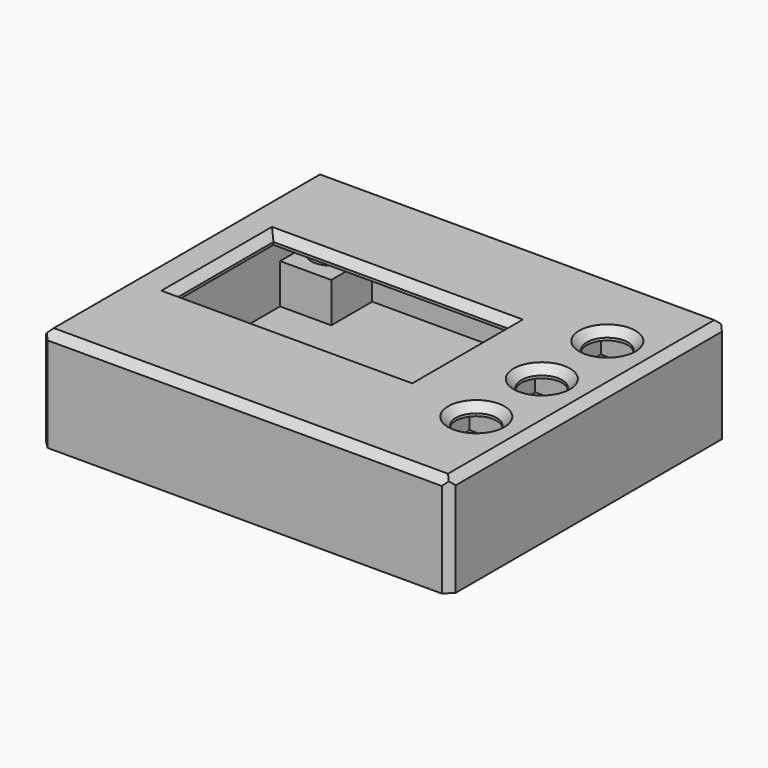
from build123d import *

# Parameters (mm, degrees)
F0_W      = 40
F0_H      = 34
F1_DEPTH  = 10
F2_W      = 37.9
F2_H      = 31.9
F3_DEPTH  = 9
F4_R      = 2
F4_W      = 23
F4_H      = 12
F5_DEPTH  = 25
F6_W      = 6.4
F6_H      = 6.4
F7_DEPTH  = 2.5
F6_W_2    = 5
F6_H_2    = 3.5
F8_DEPTH  = 1.5
F9_DEPTH  = 4
F10_R     = 1.05
F11_DEPTH = 2
F12_SIZE  = 0.75
F14_DEPTH = 2.5
F15_W     = 2
F15_H     = 2.5
F16_DEPTH = 1.1
F17_SIZE  = 0.75
F18_W     = 4.5
F18_H     = 3.5
F19_W     = 4.5
F19_H     = 3.5
F20_DEPTH = 5
F21_W     = 4.5
F21_H     = 3.5
F22_DEPTH = 4
F23_R     = 1.05
F24_R     = 1.05
F25_R     = 1.05
F26_DEPTH = 4
F27_W     = 37.5
F27_H     = 31.5
F28_DEPTH = 1.05
F29_W     = 18.5
F29_H     = 2.5
F30_DEPTH = 25
F32_R     = 1.05
F33_DEPTH = 2.95
F31_R     = 1.05
F34_DEPTH = 2.95
F35_R     = 1.05
F36_DEPTH = 2.95
F38_START = 1.6
F37_R     = 1.05
F38_DEPTH = 4.85
F39_W     = 5
F39_H     = 5
F40_DEPTH = 2
F41_W     = 5
F41_H     = 5
F42_DEPTH = 1.9
F43_DEPTH = 25
F44_R     = 1.05
F45_DEPTH = 2.1
F46_W     = 18.5
F46_H     = 1.5
F47_DEPTH = 1.5


with BuildPart() as f1:
    # F0 (on Top) → F1 (new body)
    with BuildSketch(Plane.XY):
        Rectangle(F0_W, F0_H)
    extrude(amount=F1_DEPTH)

    # F2 (on face) → F3 (cut)
    with BuildSketch(Plane(origin=(0, 0, 0), x_dir=(1, 0, 0), z_dir=(0, 0, -1))):
        Rectangle(F2_W, F2_H)
    extrude(amount=-F3_DEPTH, mode=Mode.SUBTRACT)

    # F4 (on face) → F5 (cut)
    with BuildSketch(Plane.XY.offset(10)):
        with Locations((15.05, -7.55)):
            Circle(F4_R)
        with Locations((15.05, 0.45)):
            Circle(F4_R)
        with Locations((15.05, 8.45)):
            Circle(F4_R)
        with Locations((-4.45, 0.45)):
            Rectangle(F4_W, F4_H)
    extrude(amount=-F5_DEPTH, mode=Mode.SUBTRACT)

    # F6 (on face) → F7 (join)
    with BuildSketch(Plane(origin=(0, 0, 9), x_dir=(1, 0, 0), z_dir=(0, 0, -1))):
        Polygon((18.95, 15.95), (10.25, 15.95), (10.25, 12.45), (10.25, 8.95), (10.25, -12.45), (10.25, -15.95), (18.95, -15.95), align=None)
        with Locations((15.05, -8.45)):
            Rectangle(F6_W, F6_H, mode=Mode.SUBTRACT)
        with Locations((15.05, -0.45)):
            Rectangle(F6_W, F6_H, mode=Mode.SUBTRACT)
        with Locations((15.05, 7.55)):
            Rectangle(F6_W, F6_H, mode=Mode.SUBTRACT)
    extrude(amount=F7_DEPTH)

    # F6 (on face) → F8 (join)
    with BuildSketch(Plane(origin=(0, 0, 9), x_dir=(1, 0, 0), z_dir=(0, 0, -1))):
        with Locations((-16.45, 10.7)):
            Rectangle(F6_W_2, F6_H_2)
        with Locations((7.75, 10.7)):
            Rectangle(F6_W_2, F6_H_2)
        with Locations((-16.45, -14.2)):
            Rectangle(F6_W_2, F6_H_2)
        with Locations((7.75, -14.2)):
            Rectangle(F6_W_2, F6_H_2)
    extrude(amount=F8_DEPTH)

    # F6 (on face) → F9 (join)
    with BuildSketch(Plane(origin=(0, 0, 9), x_dir=(1, 0, 0), z_dir=(0, 0, -1))):
        Polygon((-10.25, 12.45), (-10.25, 15.95), (-18.95, 15.95), (-18.95, 12.45), (-13.95, 12.45), align=None)
    extrude(amount=F9_DEPTH)

    # F10 (on face) → F11 (cut)
    with BuildSketch(Plane(origin=(0, 0, 7.5), x_dir=(1, 0, 0), z_dir=(0, 0, -1))):
        with Locations((-16.45, -13.95)):
            Circle(F10_R)
    extrude(amount=-F11_DEPTH, mode=Mode.SUBTRACT)

    # F12
    f12_edges = [f1.edges().sort_by_distance(p)[0] for p in [
        (-20, 0, 10),
        (0, 17, 10),
        (20, 0, 10),
        (0, -17, 10),
        (-4.45, 6.45, 10),
        (7.05, 0.45, 10),
        (-4.45, -5.55, 10),
        (-15.95, 0.45, 10),
        (13.05, 8.45, 10),
        (13.05, 0.45, 10),
        (13.05, -7.55, 10),
    ]]
    chamfer(f12_edges, length=F12_SIZE)

    # F13 (on face) → F14 (join)
    with BuildSketch(Plane(origin=(0, -15.95, 0), x_dir=(-1, 0, 0), z_dir=(0, 1, 0))):
        Polygon((9.25, 0), (11.25, 0), (11.25, 5), (10.25, 5), (10.25, 9), (9.25, 9), align=None)
        Polygon((-11.25, 0), (-9.25, 0), (-9.25, 9), (-10.25, 9), (-10.25, 6.5), (-11.25, 6.5), align=None)
    extrude(amount=F14_DEPTH)

    # F15 (on face) → F16 (cut)
    with BuildSketch(Plane(origin=(0, 0, 0), x_dir=(1, 0, 0), z_dir=(0, 0, -1))):
        with Locations((-10.25, 14.7)):
            Rectangle(F15_W, F15_H)
        with Locations((10.25, 14.7)):
            Rectangle(F15_W, F15_H)
    extrude(amount=-F16_DEPTH, mode=Mode.SUBTRACT)

    # F17
    f17_edges = [f1.edges().sort_by_distance(p)[0] for p in [
        (-20, 17, 4.625),
        (20, 17, 4.625),
        (-20, -17, 4.625),
        (20, -17, 4.625),
    ]]
    chamfer(f17_edges, length=F17_SIZE)

    # F18 (on face) + F19 (on face) → F20 (join, through all)
    with BuildSketch(Plane(origin=(0, 0, 5), x_dir=(1, 0, 0), z_dir=(0, 0, -1))):
        with Locations((-16.7, 14.2)):
            Rectangle(F18_W, F18_H)
    with BuildSketch(Plane(origin=(0, 0, 6.5), x_dir=(1, 0, 0), z_dir=(0, 0, -1))):
        with Locations((16.7, 14.2)):
            Rectangle(F19_W, F19_H)
        with Locations((16.7, -14.2)):
            Rectangle(F19_W, F19_H)
    extrude(amount=F20_DEPTH)

    # F21 (on face) → F22 (cut)
    with BuildSketch(Plane(origin=(0, 0, 0), x_dir=(1, 0, 0), z_dir=(0, 0, -1))):
        with Locations((-16.7, 14.2)):
            Rectangle(F21_W, F21_H)
        with Locations((16.7, 14.2)):
            Rectangle(F21_W, F21_H)
        with Locations((16.7, -14.2)):
            Rectangle(F21_W, F21_H)
    extrude(amount=-F22_DEPTH, mode=Mode.SUBTRACT)

    # F23 (on face) + F24 (on face) + F25 (on face) → F26 (cut)
    with BuildSketch(Plane(origin=(0, 0, 4), x_dir=(1, 0, 0), z_dir=(0, 0, -1))):
        with Locations((-16.45, 13.95)):
            Circle(F23_R)
    with BuildSketch(Plane(origin=(0, 0, 4), x_dir=(1, 0, 0), z_dir=(0, 0, -1))):
        with Locations((16.45, 13.95)):
            Circle(F24_R)
    with BuildSketch(Plane(origin=(0, 0, 4), x_dir=(1, 0, 0), z_dir=(0, 0, -1))):
        with Locations((16.45, -13.95)):
            Circle(F25_R)
    extrude(amount=-F26_DEPTH, mode=Mode.SUBTRACT)


with BuildPart() as f28:
    # F27 (on face) → F28 (new body)
    with BuildSketch(Plane(origin=(0, 0, 0), x_dir=(1, 0, 0), z_dir=(0, 0, -1))):
        Rectangle(F27_W, F27_H)
    extrude(amount=-F28_DEPTH)

    # F29 (on face) → F30 (cut)
    with BuildSketch(Plane(origin=(0, 0, 1.1), x_dir=(1, 0, 0), z_dir=(0, 0, -1))):
        with Locations((0, 14.7)):
            Rectangle(F29_W, F29_H)
    extrude(amount=F30_DEPTH, mode=Mode.SUBTRACT)

    # F32 (on face) → F33 (join, through all)
    with BuildSketch(Plane(origin=(0, 0, 4), x_dir=(1, 0, 0), z_dir=(0, 0, -1))):
        with BuildLine():
            ThreePointArc((17.4449874371, 12.45), (18.0360292221, 13.0988177007), (18.25, 13.95))
            ThreePointArc((18.25, 13.95), (15.5988177007, 15.5360292221), (15.4550125629, 12.45))
            Line((15.4550125629, 12.45), (17.4449874371, 12.45))
        make_face()
        with Locations((16.45, 13.95)):
            Circle(F32_R, mode=Mode.SUBTRACT)
        with BuildLine():
            Line((17.4449874371, 12.45), (15.4550125629, 12.45))
            ThreePointArc((15.4550125629, 12.45), (16.45, 12.15), (17.4449874371, 12.45))
        make_face()
    extrude(amount=F33_DEPTH)

    # F31 (on face) → F34 (join, through all)
    with BuildSketch(Plane(origin=(0, 0, 4), x_dir=(1, 0, 0), z_dir=(0, 0, -1))):
        with BuildLine():
            ThreePointArc((-15.4550125629, 12.45), (-14.8639707779, 13.0988177007), (-14.65, 13.95))
            ThreePointArc((-14.65, 13.95), (-17.3011822993, 15.5360292221), (-17.4449874371, 12.45))
            Line((-17.4449874371, 12.45), (-15.4550125629, 12.45))
        make_face()
        with Locations((-16.45, 13.95)):
            Circle(F31_R, mode=Mode.SUBTRACT)
        with BuildLine():
            Line((-15.4550125629, 12.45), (-17.4449874371, 12.45))
            ThreePointArc((-17.4449874371, 12.45), (-16.45, 12.15), (-15.4550125629, 12.45))
        make_face()
    extrude(amount=F34_DEPTH)

    # F35 (on face) → F36 (join, through all)
    with BuildSketch(Plane(origin=(0, 0, 4), x_dir=(1, 0, 0), z_dir=(0, 0, -1))):
        with BuildLine():
            Line((15.4550125629, -12.45), (17.4449874371, -12.45))
            ThreePointArc((17.4449874371, -12.45), (16.45, -12.15), (15.4550125629, -12.45))
        make_face()
        with BuildLine():
            ThreePointArc((15.4550125629, -12.45), (15.5988177007, -15.5360292221), (18.25, -13.95))
            ThreePointArc((18.25, -13.95), (18.0360292221, -13.0988177007), (17.4449874371, -12.45))
            Line((17.4449874371, -12.45), (15.4550125629, -12.45))
        make_face()
        with Locations((16.45, -13.95)):
            Circle(F35_R, mode=Mode.SUBTRACT)
    extrude(amount=F36_DEPTH)

    # F37 (on face) → F38 (join)
    with BuildSketch(Plane(origin=(0, 0, 7.5), x_dir=(1, 0, 0), z_dir=(0, 0, -1)).offset(F38_START)):
        with BuildLine():
            Line((-17.4449874371, -12.45), (-15.4550125629, -12.45))
            ThreePointArc((-15.4550125629, -12.45), (-16.45, -12.15), (-17.4449874371, -12.45))
        make_face()
        with BuildLine():
            ThreePointArc((-17.4449874371, -12.45), (-17.3011822993, -15.5360292221), (-14.65, -13.95))
            ThreePointArc((-14.65, -13.95), (-14.8639707779, -13.0988177007), (-15.4550125629, -12.45))
            Line((-15.4550125629, -12.45), (-17.4449874371, -12.45))
        make_face()
        with Locations((-16.45, -13.95)):
            Circle(F37_R, mode=Mode.SUBTRACT)
    extrude(amount=F38_DEPTH)

    # F39 (on face) → F40 (join)
    with BuildSketch(Plane.XY.offset(1.05)):
        with Locations((-16.25, 13.25)):
            Rectangle(F39_W, F39_H)
        with Locations((16.25, 13.25)):
            Rectangle(F39_W, F39_H)
        with Locations((16.25, -13.25)):
            Rectangle(F39_W, F39_H)
        with Locations((-16.25, -13.25)):
            Rectangle(F39_W, F39_H)
    extrude(amount=F40_DEPTH)

    # F41 (on face) → F42 (join)
    with BuildSketch(Plane.XY.offset(3.05)):
        with Locations((-16.25, 13.25)):
            Rectangle(F41_W, F41_H)
    extrude(amount=F42_DEPTH)

    # F43 (cut): faces of the model
    f43_faces = [f28.faces().sort_by_distance(p)[0] for p in [
        (16.45, -13.95, 3.05),
        (-16.45, -13.95, 3.05),
        (-16.45, 13.95, 4.95),
        (16.45, 13.95, 3.05),
    ]]
    extrude(f43_faces, amount=-F43_DEPTH, mode=Mode.SUBTRACT)

    # F44 (on face) → F45 (cut)
    with BuildSketch(Plane(origin=(0, 0, 0), x_dir=(1, 0, 0), z_dir=(0, 0, -1))):
        with BuildLine():
            ThreePointArc((15.5782202113, 15.75), (15.3878228908, 12.2553673588), (18.45, 13.95))
            ThreePointArc((18.45, 13.95), (18.1446326412, 15.0121771092), (17.3217797887, 15.75))
            Line((17.3217797887, 15.75), (15.5782202113, 15.75))
        make_face()
        with Locations((16.45, 13.95)):
            Circle(F44_R, mode=Mode.SUBTRACT)
        with BuildLine():
            Line((15.5782202113, -15.75), (17.3217797887, -15.75))
            ThreePointArc((17.3217797887, -15.75), (18.1446326412, -15.0121771092), (18.45, -13.95))
            ThreePointArc((18.45, -13.95), (15.3878228908, -12.2553673588), (15.5782202113, -15.75))
        make_face()
        with Locations((16.45, -13.95)):
            Circle(F44_R, mode=Mode.SUBTRACT)
        with BuildLine():
            ThreePointArc((15.5782202113, -15.75), (16.45, -15.95), (17.3217797887, -15.75))
            Line((17.3217797887, -15.75), (15.5782202113, -15.75))
        make_face()
        with BuildLine():
            Line((-17.3217797887, -15.75), (-15.5782202113, -15.75))
            ThreePointArc((-15.5782202113, -15.75), (-14.7553673588, -15.0121771092), (-14.45, -13.95))
            ThreePointArc((-14.45, -13.95), (-17.5121771092, -12.2553673588), (-17.3217797887, -15.75))
        make_face()
        with Locations((-16.45, -13.95)):
            Circle(F44_R, mode=Mode.SUBTRACT)
        with BuildLine():
            Line((-17.3217797887, 15.75), (-15.5782202113, 15.75))
            ThreePointArc((-15.5782202113, 15.75), (-16.45, 15.95), (-17.3217797887, 15.75))
        make_face()
        with BuildLine():
            ThreePointArc((-14.45, 13.95), (-14.7553673588, 15.0121771092), (-15.5782202113, 15.75))
            Line((-15.5782202113, 15.75), (-17.3217797887, 15.75))
            ThreePointArc((-17.3217797887, 15.75), (-17.5121771092, 12.2553673588), (-14.45, 13.95))
        make_face()
        with Locations((-16.45, 13.95)):
            Circle(F44_R, mode=Mode.SUBTRACT)
    extrude(amount=-F45_DEPTH, mode=Mode.SUBTRACT)

    # F46 (on face) → F47 (join)
    with BuildSketch(Plane.XY.offset(1.05)):
        with Locations((0, -12.7)):
            Rectangle(F46_W, F46_H)
    extrude(amount=F47_DEPTH)


solid = Compound([f1.part, f28.part])
